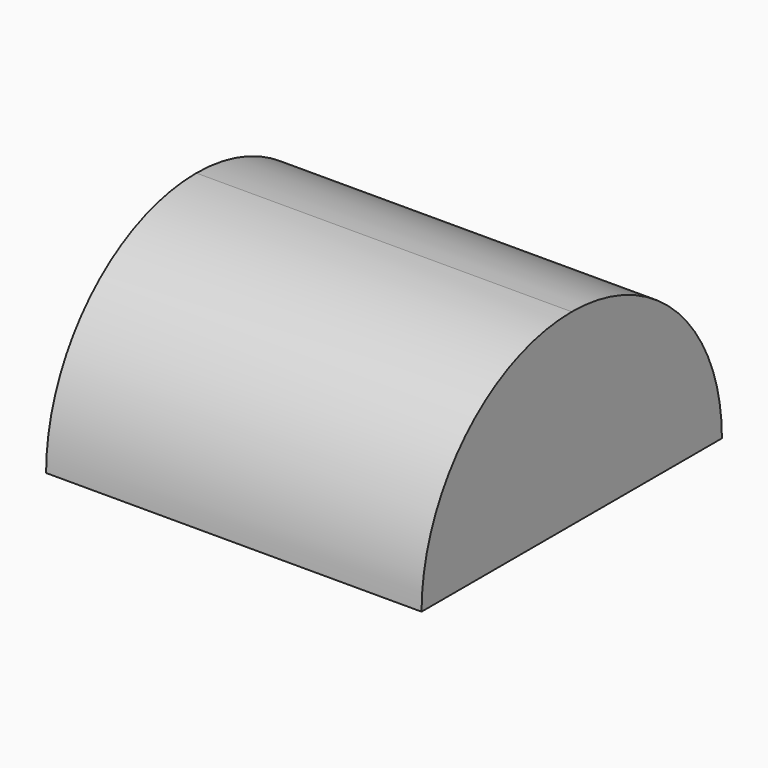
from build123d import *

# Parameters (mm, degrees)
F0_W     = 60
F0_H     = 60
F0_R     = 22.5
F1_DEPTH = 30
F2_DEPTH = 22.5
F3_R     = 22.49999
F4_R     = 29.99999


# Not quite as in the source:
# - a fillet or chamfer is up to 0.001 mm smaller than in the source, because OpenCascade refuses the exact size
# - a feature names something its author has since deleted; it is built from what else it names


with BuildPart() as f1:
    # F0 (on Top) → F1 (new body)
    with BuildSketch(Plane.XY):
        Rectangle(F0_W, F0_H)
        Circle(F0_R, mode=Mode.SUBTRACT)
        Circle(F0_R)
    extrude(amount=F1_DEPTH)

    # F0 (on Top) → F2 (cut)
    with BuildSketch(Plane.XY):
        Circle(F0_R)
    extrude(amount=F2_DEPTH, mode=Mode.SUBTRACT)

    # F3 (radius 22.5 in the source; OpenCascade refuses exactly that, so slightly less here)
    f3_edges = [f1.edges().sort_by_distance(p)[0] for p in [
        (-22.5, 0, 22.5),
    ]]
    fillet(f3_edges, radius=F3_R)

    # F4 (radius 30 in the source; OpenCascade refuses exactly that, so slightly less here)
    f4_edges = [f1.edges().sort_by_distance(p)[0] for p in [
        (0, -30, 30),
        (0, 30, 30),
    ]]
    fillet(f4_edges, radius=F4_R)


solid = f1.part
